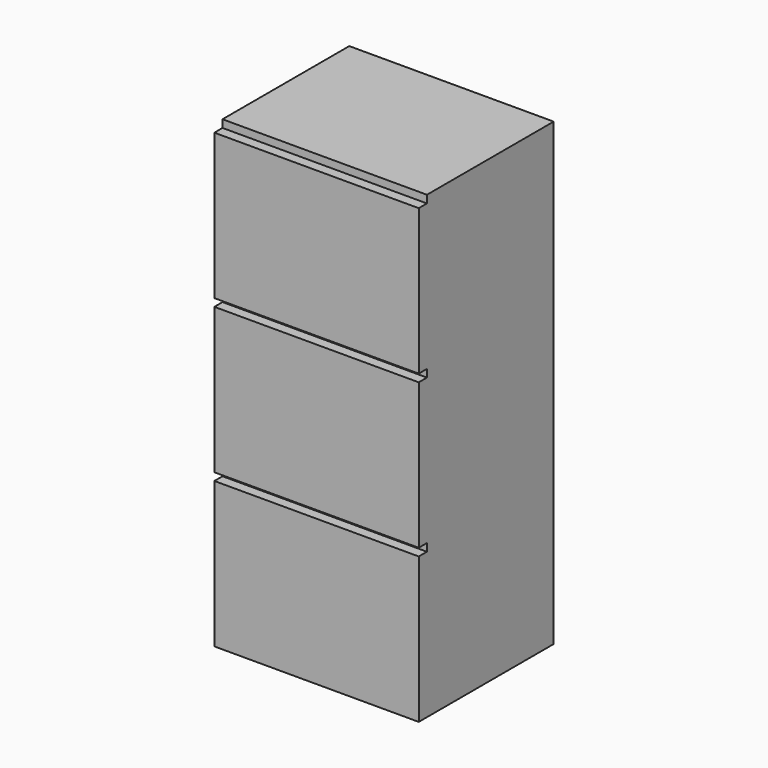
from build123d import *

# Parameters (mm, degrees)
F0_W     = 330
F0_H     = 900
F1_DEPTH = 400
F2_W     = 400
F2_H     = 15
F3_DEPTH = 20


# Not quite as in the source:
# - a feature names something its author has since deleted; it is built from what else it names


with BuildPart() as f1:
    # F0 (on Right) → F1 (new body)
    with BuildSketch(Plane.YZ):
        with Locations((165, 450)):
            Rectangle(F0_W, F0_H)
    extrude(amount=F1_DEPTH)

    # F2 (on face) → F3 (cut)
    with BuildSketch(Plane.XZ):
        with Locations((200, 892.5)):
            Rectangle(F2_W, F2_H)
        with Locations((200, 592.5)):
            Rectangle(F2_W, F2_H)
        with Locations((200, 292.5)):
            Rectangle(F2_W, F2_H)
    extrude(amount=-F3_DEPTH, mode=Mode.SUBTRACT)


solid = f1.part
